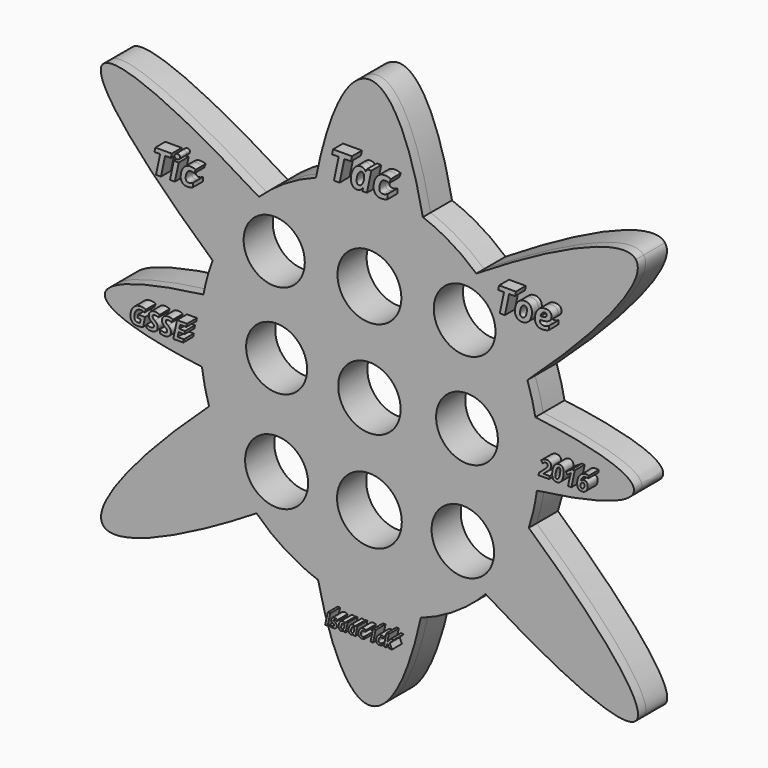
from build123d import *

# Parameters (mm, degrees)
F0_R            = 8.9206433005
F1_DEPTH        = 25.4
F3_DEPTH        = 25.4
F4_R            = 9.1284797641
F5_DEPTH        = 68.326
F6_R            = 8.5679037561
F7_DEPTH        = 25.4
F8_R            = 9.250882746
F9_DEPTH        = 72.898
F10_R           = 8.8291023819
F11_DEPTH       = 50.292
F12_R           = 8.7155706802
F13_DEPTH       = 66.548
F14_R           = 8.7386660954
F15_DEPTH       = 88.646
F16_R           = 8.8171002105
F17_DEPTH       = 41.402
F18_R           = 8.9292749257
F19_DEPTH       = 72.136
F20_R           = 8.9994513655
F21_DEPTH       = 122.936
F22_DEPTH       = 22.606
F24_DEPTH       = 1.27
F25_TEXT_SIZE   = 9.5029258066
F25_TEXT_SIZE_2 = 10.9283667472
F25_TEXT_SIZE_3 = 9.7405061954
F26_DEPTH       = 4.064
F27_TEXT_SIZE   = 7.1271966186
F27_TEXT_SIZE_2 = 6.414476795
F28_DEPTH       = 6.35
F29_TEXT_SIZE   = 4.7514680773
F30_DEPTH       = 6.35
F31_DEPTH       = 7.62
F32_DEPTH       = 6.35


# Not quite as in the source:
# - Text() gives the source's letters only with a copy of the font that has no kerning and outlines rounded to 1/6400 em; it was checked with that copy


with BuildPart() as f1:
    # F0 (on Front) → F1 (new body)
    with BuildSketch(Plane.XZ):
        with BuildLine():
            add(Edge.make_bspline(
                [(14.6742075585, -51.9117381707), (48.3704358339, -40.1372706641), (48.3704358339, -1.3252174249)],
                knots=[3.4498214843, 3.4498214843, 3.4498214843, 4.7123889804, 4.7123889804, 4.7123889804], degree=2, weights=[1, 0.8072705293, 1]))
            add(Edge.make_bspline(
                [(48.3704358339, -1.3252174249), (48.3704358339, 36.962856223), (15.2686799087, 49.0489234823)],
                knots=[4.7123889804, 4.7123889804, 4.7123889804, 5.9620316866, 5.9620316866, 5.9620316866], degree=2, weights=[1, 0.8110676324, 1]))
            add(Edge.make_bspline(
                [(14.6742075585, -51.9117381707), (25.4538410141, -2.4336206724), (15.2686799087, 49.0489234823)],
                knots=[3.9919122168, 3.9919122168, 3.9919122168, 5.3854210081, 5.3854210081, 5.3854210081], degree=2, weights=[1, 0.766929031, 1]))
        make_face()
        with BuildLine():
            add(Edge.make_bspline(
                [(14.6742075585, -51.9117381707), (25.4538410141, -2.4336206724), (15.2686799087, 49.0489234823)],
                knots=[3.9919122168, 3.9919122168, 3.9919122168, 5.3854210081, 5.3854210081, 5.3854210081], degree=2, weights=[1, 0.766929031, 1]))
            add(Edge.make_bspline(
                [(15.2686799087, 49.0489234823), (0, 54.623802735), (-15.2686799087, 49.0489234823)],
                knots=[5.9620316866, 5.9620316866, 5.9620316866, 6.6043389278, 6.6043389278, 6.6043389278], degree=2, weights=[1, 0.9488718961, 1]))
            add(Edge.make_bspline(
                [(-15.2686799087, 49.0489234823), (-25.4538410141, -2.4336206724), (-14.6742075585, -51.9117381707)],
                knots=[0.8977642991, 0.8977642991, 0.8977642991, 2.2912730904, 2.2912730904, 2.2912730904], degree=2, weights=[1, 0.766929031, 1]))
            add(Edge.make_bspline(
                [(-14.6742075585, -51.9117381707), (0, -57.0393441053), (14.6742075585, -51.9117381707)],
                knots=[2.8333638228, 2.8333638228, 2.8333638228, 3.4498214843, 3.4498214843, 3.4498214843], degree=2, weights=[1, 0.9528723863, 1]))
        make_face()
        with Locations((0, -1.3252174249)):
            Circle(F0_R, mode=Mode.SUBTRACT)
        with BuildLine():
            add(Edge.make_bspline(
                [(15.2686799087, 49.0489234823), (0, 54.623802735), (-15.2686799087, 49.0489234823)],
                knots=[5.9620316866, 5.9620316866, 5.9620316866, 6.6043389278, 6.6043389278, 6.6043389278], degree=2, weights=[1, 0.9488718961, 1]))
            add(Edge.make_bspline(
                [(15.2686799087, 49.0489234823), (9.4056048871, 78.684784472), (0, 78.684784472)],
                knots=[5.3854210081, 5.3854210081, 5.3854210081, 6.2831853072, 6.2831853072, 6.2831853072], degree=2, weights=[1, 0.9009327661, 1]))
            add(Edge.make_bspline(
                [(0, 78.684784472), (-9.4056048871, 78.684784472), (-15.2686799087, 49.0489234823)],
                knots=[0, 0, 0, 0.8977642991, 0.8977642991, 0.8977642991], degree=2, weights=[1, 0.9009327661, 1]))
        make_face()
        with BuildLine():
            add(Edge.make_bspline(
                [(-14.6742075585, -51.9117381707), (0, -119.2658062624), (14.6742075585, -51.9117381707)],
                knots=[2.2912730904, 2.2912730904, 2.2912730904, 3.9919122168, 3.9919122168, 3.9919122168], degree=2, weights=[1, 0.6597430306, 1]))
            add(Edge.make_bspline(
                [(-14.6742075585, -51.9117381707), (0, -57.0393441053), (14.6742075585, -51.9117381707)],
                knots=[2.8333638228, 2.8333638228, 2.8333638228, 3.4498214843, 3.4498214843, 3.4498214843], degree=2, weights=[1, 0.9528723863, 1]))
        make_face()
        with BuildLine():
            add(Edge.make_bspline(
                [(-15.2686799087, 49.0489234823), (-25.4538410141, -2.4336206724), (-14.6742075585, -51.9117381707)],
                knots=[0.8977642991, 0.8977642991, 0.8977642991, 2.2912730904, 2.2912730904, 2.2912730904], degree=2, weights=[1, 0.766929031, 1]))
            add(Edge.make_bspline(
                [(-15.2686799087, 49.0489234823), (-156.270924432, -2.4336206724), (-14.6742075585, -51.9117381707)],
                knots=[0.3211536206, 0.3211536206, 0.3211536206, 2.8333638228, 2.8333638228, 2.8333638228], degree=2, weights=[1, 0.3095228749, 1]))
        make_face()
    extrude(amount=F1_DEPTH)

    # F2 (on Front) → F3 (join)
    with BuildSketch(Plane.XZ):
        with BuildLine():
            add(Edge.make_bspline(
                [(-35.3874231798, 10.428298438), (-75.6044536829, 7.1034550323), (-75.6044536829, 0)],
                knots=[5.1994831942, 5.1994831942, 5.1994831942, 6.2831853072, 6.2831853072, 6.2831853072], degree=2, weights=[1, 0.8567555177, 1]))
            add(Edge.make_bspline(
                [(-75.6044536829, 0), (-75.6044536829, -6.9397754477), (-36.7486800422, -10.3129575167)],
                knots=[0, 0, 0, 1.0632149091, 1.0632149091, 1.0632149091], degree=2, weights=[1, 0.8619933343, 1]))
            add(Edge.make_bspline(
                [(-23.6245814509, 0.7197530422), (-30.4510036643, -4.8386106263), (-36.7486800422, -10.3129575167)],
                knots=[1.7633892798, 1.7633892798, 1.7633892798, 1.9500135403, 1.9500135403, 1.9500135403], degree=2, weights=[1, 0.9956495812, 1]))
            add(Edge.make_bspline(
                [(-35.3874231798, 10.428298438), (-29.7109719827, 5.6127468854), (-23.6245814509, 0.7197530422)],
                knots=[1.2014332241, 1.2014332241, 1.2014332241, 1.3677426954, 1.3677426954, 1.3677426954], degree=2, weights=[1, 0.9965446367, 1]))
        make_face()
        with BuildLine():
            add(Edge.make_bspline(
                [(-23.6245814509, 0.7197530422), (-30.4510036643, -4.8386106263), (-36.7486800422, -10.3129575167)],
                knots=[1.7633892798, 1.7633892798, 1.7633892798, 1.9500135403, 1.9500135403, 1.9500135403], degree=2, weights=[1, 0.9956495812, 1]))
            add(Edge.make_bspline(
                [(-36.7486800422, -10.3129575167), (-23.1218635797, -11.4959408584), (-7.6083152612, -11.7408614978)],
                knots=[1.0632149091, 1.0632149091, 1.0632149091, 1.4699925331, 1.4699925331, 1.4699925331], degree=2, weights=[1, 0.9793876986, 1]))
            add(Edge.make_bspline(
                [(-23.6245814509, 0.7197530422), (-15.7959283164, -5.5738870697), (-7.6083152612, -11.7408614978)],
                knots=[1.3677426954, 1.3677426954, 1.3677426954, 1.5813377968, 1.5813377968, 1.5813377968], degree=2, weights=[1, 0.9943025599, 1]))
        make_face()
        with BuildLine():
            add(Edge.make_bspline(
                [(-36.7486800422, -10.3129575167), (-23.1218635797, -11.4959408584), (-7.6083152612, -11.7408614978)],
                knots=[1.0632149091, 1.0632149091, 1.0632149091, 1.4699925331, 1.4699925331, 1.4699925331], degree=2, weights=[1, 0.9793876986, 1]))
            add(Edge.make_bspline(
                [(-36.7486800422, -10.3129575167), (-89.4088868265, -56.0886090359), (-74.1556971976, -59.2603531034), (-58.9025075688, -62.4320971709), (1.09197667, -18.1815332938)],
                knots=[1.9500135403, 1.9500135403, 1.9500135403, 3.2780135851, 3.2780135851, 4.6060136299, 4.6060136299, 4.6060136299], degree=2, weights=[1, 0.7875334369, 1, 0.7875334369, 1]))
            add(Edge.make_bspline(
                [(-7.6083152612, -11.7408614978), (-3.2686888516, -15.0095021767), (1.09197667, -18.1815332938)],
                knots=[1.5813377968, 1.5813377968, 1.5813377968, 1.6948585155, 1.6948585155, 1.6948585155], degree=2, weights=[1, 0.9983895632, 1]))
        make_face()
        with BuildLine():
            add(Edge.make_bspline(
                [(-76.2886628509, 57.6453916728), (-82.0531350574, 50.0166140045), (-35.3874231798, 10.428298438)],
                knots=[0, 0, 0, 1.2014332241, 1.2014332241, 1.2014332241], degree=2, weights=[1, 0.8249307734, 1]))
            add(Edge.make_bspline(
                [(-9.7120202802, 11.7029965146), (-23.2891359116, 11.4284943784), (-35.3874231798, 10.428298438)],
                knots=[4.8412032322, 4.8412032322, 4.8412032322, 5.1994831942, 5.1994831942, 5.1994831942], degree=2, weights=[1, 0.9839972978, 1]))
            add(Edge.make_bspline(
                [(-1.09197667, 18.1815332938), (-5.4192075972, 14.98986641), (-9.7120202802, 11.7029965146)],
                knots=[1.4644209763, 1.4644209763, 1.4644209763, 1.5771852649, 1.5771852649, 1.5771852649], degree=2, weights=[1, 0.9984109479, 1]))
            add(Edge.make_bspline(
                [(-1.09197667, 18.1815332938), (-68.8596573723, 67.4770343736), (-76.2886628509, 57.6453916728)],
                knots=[4.8364511691, 4.8364511691, 4.8364511691, 6.2831853072, 6.2831853072, 6.2831853072], degree=2, weights=[1, 0.749581278, 1]))
        make_face()
        with BuildLine():
            add(Edge.make_bspline(
                [(-9.7120202802, 11.7029965146), (-23.2891359116, 11.4284943784), (-35.3874231798, 10.428298438)],
                knots=[4.8412032322, 4.8412032322, 4.8412032322, 5.1994831942, 5.1994831942, 5.1994831942], degree=2, weights=[1, 0.9839972978, 1]))
            add(Edge.make_bspline(
                [(-35.3874231798, 10.428298438), (-29.7109719827, 5.6127468854), (-23.6245814509, 0.7197530422)],
                knots=[1.2014332241, 1.2014332241, 1.2014332241, 1.3677426954, 1.3677426954, 1.3677426954], degree=2, weights=[1, 0.9965446367, 1]))
            add(Edge.make_bspline(
                [(-9.7120202802, 11.7029965146), (-16.8136204503, 6.2655275328), (-23.6245814509, 0.7197530422)],
                knots=[1.5771852649, 1.5771852649, 1.5771852649, 1.7633892798, 1.7633892798, 1.7633892798], degree=2, weights=[1, 0.9956691378, 1]))
        make_face()
        with BuildLine():
            add(Edge.make_bspline(
                [(-7.6083152612, -11.7408614978), (1.065839845, -11.8778049985), (9.7120202802, -11.7029965146)],
                knots=[1.4699925331, 1.4699925331, 1.4699925331, 1.6996105787, 1.6996105787, 1.6996105787], degree=2, weights=[1, 0.9934166802, 1]))
            add(Edge.make_bspline(
                [(-7.6083152612, -11.7408614978), (-3.2686888516, -15.0095021767), (1.09197667, -18.1815332938)],
                knots=[1.5813377968, 1.5813377968, 1.5813377968, 1.6948585155, 1.6948585155, 1.6948585155], degree=2, weights=[1, 0.9983895632, 1]))
            add(Edge.make_bspline(
                [(1.09197667, -18.1815332938), (5.4192075972, -14.98986641), (9.7120202802, -11.7029965146)],
                knots=[4.6060136299, 4.6060136299, 4.6060136299, 4.7187779184, 4.7187779184, 4.7187779184], degree=2, weights=[1, 0.9984109479, 1]))
        make_face()
        with BuildLine():
            add(Edge.make_bspline(
                [(1.09197667, -18.1815332938), (5.4192075972, -14.98986641), (9.7120202802, -11.7029965146)],
                knots=[4.6060136299, 4.6060136299, 4.6060136299, 4.7187779184, 4.7187779184, 4.7187779184], degree=2, weights=[1, 0.9984109479, 1]))
            add(Edge.make_bspline(
                [(1.09197667, -18.1815332938), (60.9043687572, -61.6902059851), (74.6863029221, -58.5744987055), (88.4682370869, -55.4587914259), (35.3874231798, -10.428298438)],
                knots=[1.6948585155, 1.6948585155, 1.6948585155, 3.0189421966, 3.0189421966, 4.3430258777, 4.3430258777, 4.3430258777], degree=2, weights=[1, 0.7887386987, 1, 0.7887386987, 1]))
            add(Edge.make_bspline(
                [(9.7120202802, -11.7029965146), (23.2891359116, -11.4284943784), (35.3874231798, -10.428298438)],
                knots=[1.6996105787, 1.6996105787, 1.6996105787, 2.0578905406, 2.0578905406, 2.0578905406], degree=2, weights=[1, 0.9839972978, 1]))
        make_face()
        with BuildLine():
            add(Edge.make_bspline(
                [(-1.09197667, 18.1815332938), (-5.4192075972, 14.98986641), (-9.7120202802, 11.7029965146)],
                knots=[1.4644209763, 1.4644209763, 1.4644209763, 1.5771852649, 1.5771852649, 1.5771852649], degree=2, weights=[1, 0.9984109479, 1]))
            add(Edge.make_bspline(
                [(7.6083152612, 11.7408614978), (-1.065839845, 11.8778049985), (-9.7120202802, 11.7029965146)],
                knots=[4.6115851867, 4.6115851867, 4.6115851867, 4.8412032322, 4.8412032322, 4.8412032322], degree=2, weights=[1, 0.9934166802, 1]))
            add(Edge.make_bspline(
                [(7.6083152612, 11.7408614978), (3.2686888516, 15.0095021767), (-1.09197667, 18.1815332938)],
                knots=[4.7229304504, 4.7229304504, 4.7229304504, 4.8364511691, 4.8364511691, 4.8364511691], degree=2, weights=[1, 0.9983895632, 1]))
        make_face()
        with BuildLine():
            add(Edge.make_bspline(
                [(9.7120202802, -11.7029965146), (16.8136204503, -6.2655275328), (23.6245814509, -0.7197530422)],
                knots=[4.7187779184, 4.7187779184, 4.7187779184, 4.9049819334, 4.9049819334, 4.9049819334], degree=2, weights=[1, 0.9956691378, 1]))
            add(Edge.make_bspline(
                [(9.7120202802, -11.7029965146), (23.2891359116, -11.4284943784), (35.3874231798, -10.428298438)],
                knots=[1.6996105787, 1.6996105787, 1.6996105787, 2.0578905406, 2.0578905406, 2.0578905406], degree=2, weights=[1, 0.9839972978, 1]))
            add(Edge.make_bspline(
                [(35.3874231798, -10.428298438), (29.7109719827, -5.6127468854), (23.6245814509, -0.7197530422)],
                knots=[4.3430258777, 4.3430258777, 4.3430258777, 4.5093353489, 4.5093353489, 4.5093353489], degree=2, weights=[1, 0.9965446367, 1]))
        make_face()
        with BuildLine():
            add(Edge.make_bspline(
                [(35.3874231798, -10.428298438), (29.7109719827, -5.6127468854), (23.6245814509, -0.7197530422)],
                knots=[4.3430258777, 4.3430258777, 4.3430258777, 4.5093353489, 4.5093353489, 4.5093353489], degree=2, weights=[1, 0.9965446367, 1]))
            add(Edge.make_bspline(
                [(35.3874231798, -10.428298438), (158.4625004985, -0.2533711968), (36.7486800422, 10.3129575167)],
                knots=[2.0578905406, 2.0578905406, 2.0578905406, 4.2048075627, 4.2048075627, 4.2048075627], degree=2, weights=[1, 0.477087556, 1]))
            add(Edge.make_bspline(
                [(23.6245814509, -0.7197530422), (30.4510036643, 4.8386106263), (36.7486800422, 10.3129575167)],
                knots=[4.9049819334, 4.9049819334, 4.9049819334, 5.0916061938, 5.0916061938, 5.0916061938], degree=2, weights=[1, 0.9956495812, 1]))
        make_face()
        with BuildLine():
            add(Edge.make_bspline(
                [(7.6083152612, 11.7408614978), (3.2686888516, 15.0095021767), (-1.09197667, 18.1815332938)],
                knots=[4.7229304504, 4.7229304504, 4.7229304504, 4.8364511691, 4.8364511691, 4.8364511691], degree=2, weights=[1, 0.9983895632, 1]))
            add(Edge.make_bspline(
                [(36.7486800422, 10.3129575167), (23.1218635797, 11.4959408584), (7.6083152612, 11.7408614978)],
                knots=[4.2048075627, 4.2048075627, 4.2048075627, 4.6115851867, 4.6115851867, 4.6115851867], degree=2, weights=[1, 0.9793876986, 1]))
            add(Edge.make_bspline(
                [(36.7486800422, 10.3129575167), (82.3725207089, 49.9721453334), (76.1176049709, 58.1585466862)],
                knots=[5.0916061938, 5.0916061938, 5.0916061938, 6.2831853072, 6.2831853072, 6.2831853072], degree=2, weights=[1, 0.8277056873, 1]))
            add(Edge.make_bspline(
                [(76.1176049709, 58.1585466862), (67.8243847559, 69.0126703917), (-1.09197667, 18.1815332938)],
                knots=[0, 0, 0, 1.4644209763, 1.4644209763, 1.4644209763], degree=2, weights=[1, 0.7436984756, 1]))
        make_face()
        with BuildLine():
            add(Edge.make_bspline(
                [(36.7486800422, 10.3129575167), (23.1218635797, 11.4959408584), (7.6083152612, 11.7408614978)],
                knots=[4.2048075627, 4.2048075627, 4.2048075627, 4.6115851867, 4.6115851867, 4.6115851867], degree=2, weights=[1, 0.9793876986, 1]))
            add(Edge.make_bspline(
                [(23.6245814509, -0.7197530422), (15.7959283164, 5.5738870697), (7.6083152612, 11.7408614978)],
                knots=[4.5093353489, 4.5093353489, 4.5093353489, 4.7229304504, 4.7229304504, 4.7229304504], degree=2, weights=[1, 0.9943025599, 1]))
            add(Edge.make_bspline(
                [(23.6245814509, -0.7197530422), (30.4510036643, 4.8386106263), (36.7486800422, 10.3129575167)],
                knots=[4.9049819334, 4.9049819334, 4.9049819334, 5.0916061938, 5.0916061938, 5.0916061938], degree=2, weights=[1, 0.9956495812, 1]))
        make_face()
    extrude(amount=F3_DEPTH)

    # F4 (on Front) → F5 (cut)
    with BuildSketch(Plane.XZ):
        with Locations((0, 26.6851950437)):
            Circle(F4_R)
    extrude(amount=F5_DEPTH, mode=Mode.SUBTRACT)

    # F6 (on Front) → F7 (cut)
    with BuildSketch(Plane.XZ):
        with Locations((0, -28.9020016789)):
            Circle(F6_R)
    extrude(amount=-F7_DEPTH, mode=Mode.SUBTRACT)

    # F8 (on Front) → F9 (cut)
    with BuildSketch(Plane.XZ):
        with Locations((0, -29.5905191451)):
            Circle(F8_R)
    extrude(amount=F9_DEPTH, mode=Mode.SUBTRACT)

    # F10 (on Front) → F11 (cut)
    with BuildSketch(Plane.XZ):
        with Locations((27.8809219599, 0)):
            Circle(F10_R)
    extrude(amount=F11_DEPTH, mode=Mode.SUBTRACT)

    # F12 (on Front) → F13 (cut)
    with BuildSketch(Plane.XZ):
        with Locations((-26.5131518245, 0)):
            Circle(F12_R)
    extrude(amount=F13_DEPTH, mode=Mode.SUBTRACT)

    # F14 (on Front) → F15 (cut)
    with BuildSketch(Plane.XZ):
        with Locations((-27.1973833442, 26.6851875931)):
            Circle(F14_R)
    extrude(amount=F15_DEPTH, mode=Mode.SUBTRACT)

    # F16 (on Front) → F17 (cut)
    with BuildSketch(Plane.XZ):
        with Locations((27.1970611066, 27.0266830921)):
            Circle(F16_R)
    extrude(amount=F17_DEPTH, mode=Mode.SUBTRACT)

    # F18 (on Front) → F19 (cut)
    with BuildSketch(Plane.XZ):
        with Locations((26.6840886325, -28.7370514125)):
            Circle(F18_R)
    extrude(amount=F19_DEPTH, mode=Mode.SUBTRACT)

    # F20 (on Front) → F21 (cut)
    with BuildSketch(Plane.XZ):
        with Locations((-26.5134032816, -28.5659972578)):
            Circle(F20_R)
    extrude(amount=F21_DEPTH, mode=Mode.SUBTRACT)

    # F22 (cut): a face of the model
    f22_faces = [f1.faces().sort_by_distance(p)[0] for p in [
        (2.155e-07, -25.4, -76.4864184101),
    ]]
    extrude(f22_faces, amount=-F22_DEPTH, mode=Mode.SUBTRACT)

    # F23 (on Front) → F24 (cut)
    with BuildSketch(Plane.XZ):
        Polygon((-56.2759451568, 49.6060103178), (-67.3942342401, 49.6060103178), (-67.3942342401, 48.5797040164), (-61.8350896984, 48.5797040164), (-56.2759451568, 48.5797040164), align=None)
    extrude(amount=-F24_DEPTH, mode=Mode.SUBTRACT)

    # F25 (on Front) → F26 (join)
    with BuildSketch(Plane.XZ):
        with Locations((-59.3555904925, 37.2898578644)):
            Text('Tic', F25_TEXT_SIZE, font='Open Sans', font_style=FontStyle.BOLDITALIC, text_align=(TextAlign.LEFT, TextAlign.BOTTOM))
        with Locations((-8.7239826098, 52.3424968123)):
            Text('Tac', F25_TEXT_SIZE_2, font='Open Sans', font_style=FontStyle.BOLDITALIC, text_align=(TextAlign.LEFT, TextAlign.BOTTOM))
        with Locations((38.8289839029, 34.3819595873)):
            Text('Toe', F25_TEXT_SIZE_3, font='Open Sans', font_style=FontStyle.BOLDITALIC, text_align=(TextAlign.LEFT, TextAlign.BOTTOM))
    extrude(amount=F26_DEPTH)

    # F27 (on Front) → F28 (join)
    with BuildSketch(Plane.XZ):
        with Locations((-65.8553987741, -2.394373063)):
            Text('GSSE', F27_TEXT_SIZE, font='Open Sans', font_style=FontStyle.BOLDITALIC, text_align=(TextAlign.LEFT, TextAlign.BOTTOM))
        with Locations((51.3157062232, -2.7364783455)):
            Text('2016', F27_TEXT_SIZE_2, font='Open Sans', font_style=FontStyle.BOLDITALIC, text_align=(TextAlign.LEFT, TextAlign.BOTTOM))
    extrude(amount=F28_DEPTH)

    # F29 (on Front) → F30 (join)
    with BuildSketch(Plane.XZ):
        with Locations((-9.9210385233, -60.2101907134)):
            Text('Isaac Ick', F29_TEXT_SIZE, font='Open Sans', font_style=FontStyle.BOLDITALIC, text_align=(TextAlign.LEFT, TextAlign.BOTTOM))
    extrude(amount=F30_DEPTH)

    # F31 (add): a face of the model
    f31_faces = [f1.faces().sort_by_distance(p)[0] for p in [
        (2.155e-07, 0, -76.4864184101),
    ]]
    extrude(f31_faces, amount=F31_DEPTH)

    # F25 (on Front) → F32 (join)
    with BuildSketch(Plane.XZ):
        with Locations((-59.3555904925, 37.2898578644)):
            Text('Tic', F25_TEXT_SIZE, font='Open Sans', font_style=FontStyle.BOLDITALIC, text_align=(TextAlign.LEFT, TextAlign.BOTTOM))
        with Locations((-8.7239826098, 52.3424968123)):
            Text('Tac', F25_TEXT_SIZE_2, font='Open Sans', font_style=FontStyle.BOLDITALIC, text_align=(TextAlign.LEFT, TextAlign.BOTTOM))
        with Locations((38.8289839029, 34.3819595873)):
            Text('Toe', F25_TEXT_SIZE_3, font='Open Sans', font_style=FontStyle.BOLDITALIC, text_align=(TextAlign.LEFT, TextAlign.BOTTOM))
    extrude(amount=F32_DEPTH)


solid = f1.part
